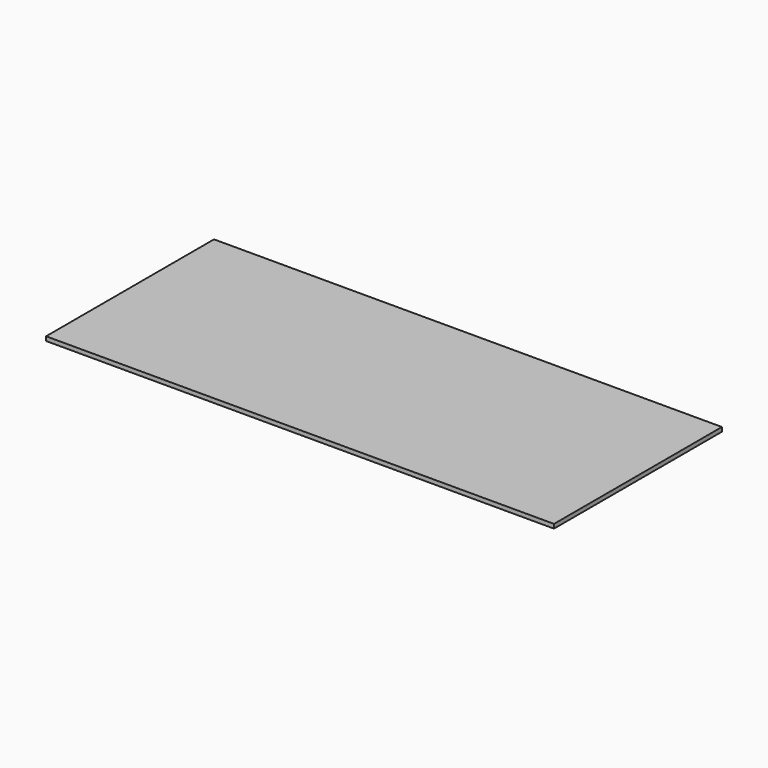
from build123d import *

# Parameters (mm, degrees)
F0_W     = 1536.7
F0_H     = 635
F2_DEPTH = 12.7


# Not quite as in the source:
# - a variable given as a bare number and used for a length is read in inches; the dataset says mm whatever the document's units were


with BuildPart() as f2:
    # F0 (on Top) → F2 (new body)
    with BuildSketch(Plane.XY):
        Rectangle(F0_W, F0_H)
    extrude(amount=F2_DEPTH)


solid = f2.part
